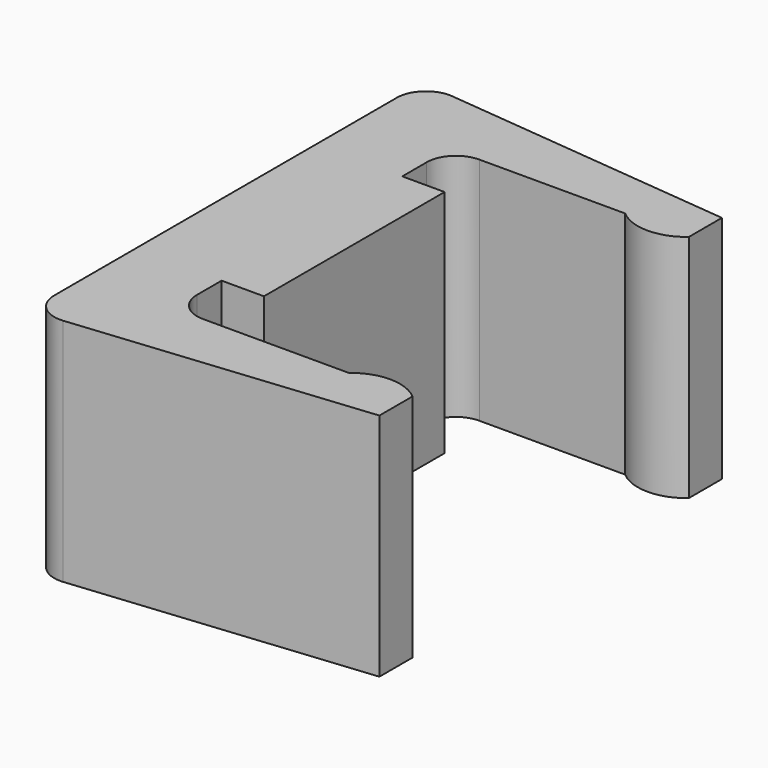
from build123d import *

# Parameters (mm, degrees)
F1_DEPTH = 50


# Not quite as in the source:
# - a feature names something its author has since deleted; it is built from what else it names


with BuildPart() as f1:
    # F0 (on Top) → F1 (new body)
    with BuildSketch(Plane.XY):
        Polygon((-28, 24.552706346), (-28, 0), (0, 0), (0, 24.552706346), (-9.2052005051, 24.552706346), align=None)
        with BuildLine():
            Line((-28, 46.552706346), (-28, 24.552706346))
            Line((-28, 24.552706346), (-9.2052005051, 24.552706346))
            Line((-9.2052005051, 24.552706346), (-9.2052005051, 31.202706346))
            ThreePointArc((-9.2052005051, 31.202706346), (-7.3453285656, 35.6928344065), (-2.8552005051, 37.552706346))
            Line((-2.8552005051, 37.552706346), (28.8586538925, 37.552706346))
            Line((28.8586538925, 37.552706346), (42.7064734879, 37.552706346))
            Line((42.7064734879, 37.552706346), (42.7064734879, 46.552706346))
            Line((42.7064734879, 46.552706346), (-28, 46.552706346))
        make_face()
        with BuildLine():
            ThreePointArc((28.8586538925, 37.552706346), (35.7825636902, 35), (42.7064734879, 37.552706346))
            Line((42.7064734879, 37.552706346), (28.8586538925, 37.552706346))
        make_face()
        with BuildLine():
            ThreePointArc((-21.0234507531, 52.8717201964), (-25.9128577435, 51.2591427749), (-28, 46.552706346))
            Line((-28, 46.552706346), (42.7064734879, 46.552706346))
            Line((42.7064734879, 46.552706346), (-21.0234507531, 52.8717201964))
        make_face()
        Polygon((0, 0), (-28, 0), (-28, -24.552706346), (-9.2052005051, -24.552706346), (0, -24.552706346), align=None)
        with BuildLine():
            Line((-9.2052005051, -24.552706346), (-28, -24.552706346))
            Line((-28, -24.552706346), (-28, -46.552706346))
            Line((-28, -46.552706346), (42.7064734879, -46.552706346))
            Line((42.7064734879, -46.552706346), (42.7064734879, -37.552706346))
            Line((42.7064734879, -37.552706346), (28.8586538925, -37.552706346))
            Line((28.8586538925, -37.552706346), (-2.8552005051, -37.552706346))
            ThreePointArc((-2.8552005051, -37.552706346), (-7.3453285656, -35.6928344065), (-9.2052005051, -31.202706346))
            Line((-9.2052005051, -31.202706346), (-9.2052005051, -24.552706346))
        make_face()
        with BuildLine():
            Line((42.7064734879, -46.552706346), (-28, -46.552706346))
            ThreePointArc((-28, -46.552706346), (-25.9128577435, -51.2591427749), (-21.0234507531, -52.8717201964))
            Line((-21.0234507531, -52.8717201964), (42.7064734879, -46.552706346))
        make_face()
        with BuildLine():
            Line((28.8586538925, -37.552706346), (42.7064734879, -37.552706346))
            ThreePointArc((42.7064734879, -37.552706346), (35.7825636902, -35), (28.8586538925, -37.552706346))
        make_face()
    extrude(amount=F1_DEPTH)


solid = f1.part
